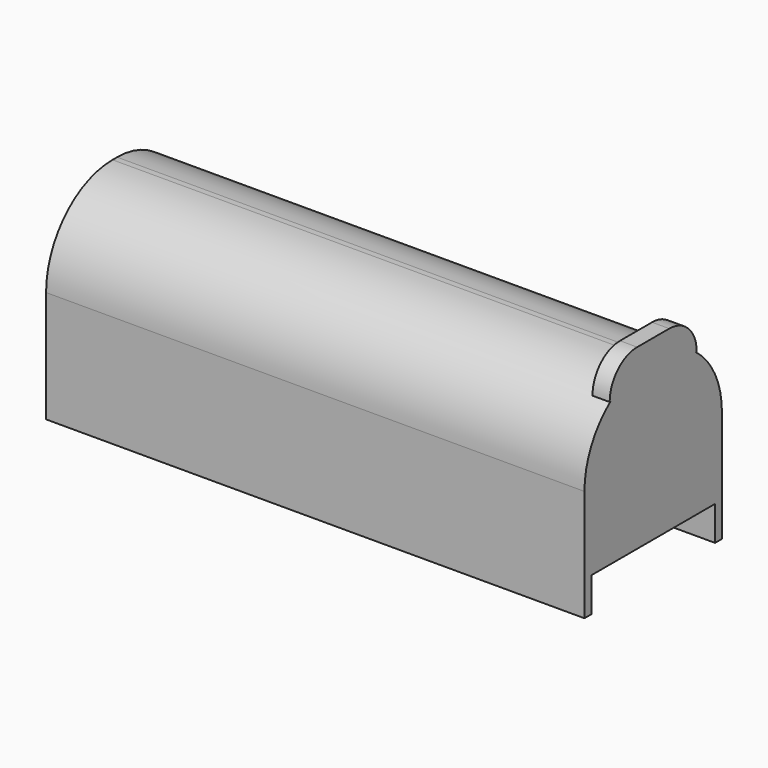
from build123d import *

# Parameters (mm, degrees)
F0_W     = 94
F0_H     = 30
F1_DEPTH = 28
F2_W     = 94
F2_H     = 1.5
F3_DEPTH = 6
F4_R     = 14.5
F6_DEPTH = 3
F7_R     = 5.99999


# Not quite as in the source:
# - a fillet or chamfer is up to 0.001 mm smaller than in the source, because OpenCascade refuses the exact size


with BuildPart() as f1:
    # F0 (on Top) → F1 (new body)
    with BuildSketch(Plane.XY):
        with Locations((47, -15)):
            Rectangle(F0_W, F0_H)
    extrude(amount=F1_DEPTH)

    # F2 (on face) → F3 (join)
    with BuildSketch(Plane(origin=(0, 0, 0), x_dir=(1, 0, 0), z_dir=(0, 0, -1))):
        with Locations((47, 0.75)):
            Rectangle(F2_W, F2_H)
        with Locations((47, 29.25)):
            Rectangle(F2_W, F2_H)
    extrude(amount=F3_DEPTH)

    # F4
    f4_edges = [f1.edges().sort_by_distance(p)[0] for p in [
        (47, 0, 28),
        (47, -30, 28),
    ]]
    fillet(f4_edges, radius=F4_R)

    # F5 (on face) → F6 (join)
    with BuildSketch(Plane.YZ.offset(94)):
        with BuildLine():
            Line((-5.5, 31), (-24.5, 31))
            Line((-24.5, 31), (-24.5, 25))
            Line((-24.5, 25), (-24.3317608663, 25))
            ThreePointArc((-24.3317608663, 25), (-20.1636895265, 27.2295302177), (-15.5, 28))
            Line((-15.5, 28), (-14.5, 28))
            ThreePointArc((-14.5, 28), (-9.8363104735, 27.2295302177), (-5.6682391337, 25))
            Line((-5.6682391337, 25), (-5.5, 25))
            Line((-5.5, 25), (-5.5, 31))
        make_face()
    extrude(amount=-F6_DEPTH)

    # F7 (radius 6 in the source; OpenCascade refuses exactly that, so slightly less here)
    f7_edges = [f1.edges().sort_by_distance(p)[0] for p in [
        (92.5, -24.5, 31),
        (92.5, -5.5, 31),
    ]]
    fillet(f7_edges, radius=F7_R)


solid = f1.part
